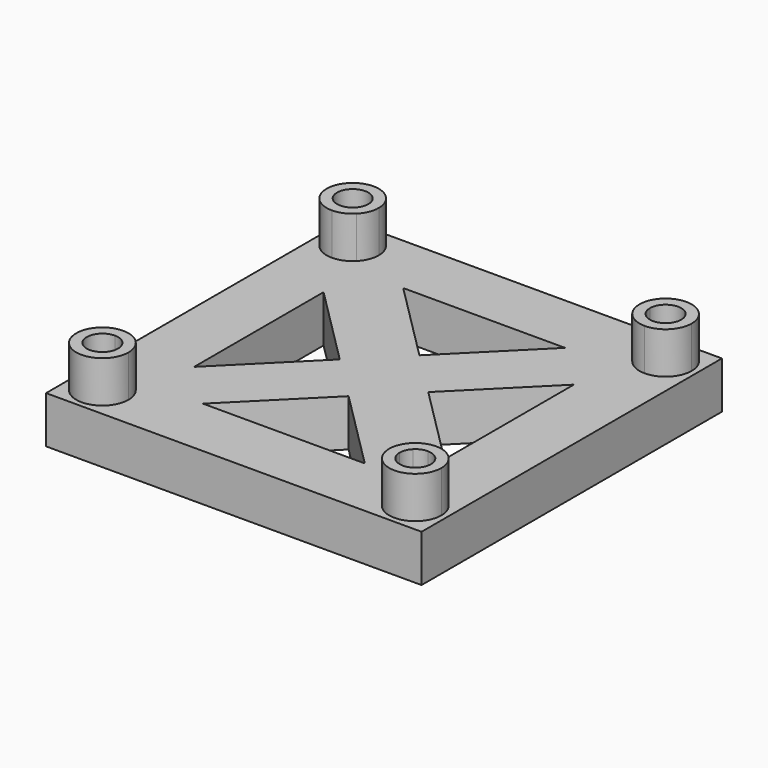
from build123d import *
from build123d import SkipClean  # not in build123d's __all__

# Parameters (mm, degrees)
F1_W     = 36
F1_H     = 36
F2_DEPTH = 4.5
F3_DEPTH = 4


with BuildPart() as f2:
    # F1 (on Top) → F2 (new body)
    with BuildSketch(Plane.XY):
        Rectangle(F1_W, F1_H)
        with BuildLine():
            ThreePointArc((-15, 12.5), (-16.767766953, 16.767766953), (-12.5, 15))
            Line((-12.5, 15), (12.5, 15))
            ThreePointArc((12.5, 15), (15, 17.5), (17.5, 15))
            ThreePointArc((17.5, 15), (16.767766953, 13.232233047), (15, 12.5))
            Line((15, 12.5), (15, -12.5))
            ThreePointArc((15, -12.5), (16.767766953, -13.232233047), (17.5, -15))
            ThreePointArc((17.5, -15), (15, -17.5), (12.5, -15))
            Line((12.5, -15), (-12.5, -15))
            ThreePointArc((-12.5, -15), (-16.767766953, -16.767766953), (-15, -12.5))
            Line((-15, -12.5), (-15, 12.5))
        make_face(mode=Mode.SUBTRACT)
        with BuildLine():
            ThreePointArc((-13.232233047, 13.232233047), (-14.0432914191, 12.6903011687), (-15, 12.5))
            Line((-15, 12.5), (-15, -12.5))
            ThreePointArc((-15, -12.5), (-14.0432914191, -12.6903011687), (-13.232233047, -13.232233047))
            Line((-13.232233047, -13.232233047), (-12, -12))
            Line((-12, -12), (-12, -7.7573593129))
            Line((-12, -7.7573593129), (-12, 7.7573593129))
            Line((-12, 7.7573593129), (-12, 12))
            Line((-12, 12), (-13.232233047, 13.232233047))
        make_face()
        with BuildLine():
            Line((12.5, 15), (-12.5, 15))
            ThreePointArc((-12.5, 15), (-12.6903011687, 14.0432914191), (-13.232233047, 13.232233047))
            Line((-13.232233047, 13.232233047), (-12, 12))
            Line((-12, 12), (-7.7573593129, 12))
            Line((-7.7573593129, 12), (7.7573593129, 12))
            Line((7.7573593129, 12), (12, 12))
            Line((12, 12), (13.232233047, 13.232233047))
            ThreePointArc((13.232233047, 13.232233047), (12.6903011687, 14.0432914191), (12.5, 15))
        make_face()
        with BuildLine():
            Line((-12, -12), (-13.232233047, -13.232233047))
            ThreePointArc((-13.232233047, -13.232233047), (-12.6903011687, -14.0432914191), (-12.5, -15))
            Line((-12.5, -15), (12.5, -15))
            ThreePointArc((12.5, -15), (12.6903011687, -14.0432914191), (13.232233047, -13.232233047))
            Line((13.232233047, -13.232233047), (12, -12))
            Line((12, -12), (7.7573593129, -12))
            Line((7.7573593129, -12), (-7.7573593129, -12))
            Line((-7.7573593129, -12), (-12, -12))
        make_face()
        with BuildLine():
            ThreePointArc((15, 12.5), (14.0432914191, 12.6903011687), (13.232233047, 13.232233047))
            Line((13.232233047, 13.232233047), (12, 12))
            Line((12, 12), (12, 7.7573593129))
            Line((12, 7.7573593129), (12, -7.7573593129))
            Line((12, -7.7573593129), (12, -12))
            Line((12, -12), (13.232233047, -13.232233047))
            ThreePointArc((13.232233047, -13.232233047), (14.0432914191, -12.6903011687), (15, -12.5))
            Line((15, -12.5), (15, 12.5))
        make_face()
        Polygon((0, 0), (-12, 12), (-12, 7.7573593129), (-4.2426406871, 0), (-2.1213203436, -2.1213203436), align=None)
        Polygon((-7.7573593129, 12), (-12, 12), (0, 0), (2.1213203436, 2.1213203436), (0, 4.2426406871), align=None)
        Polygon((2.1213203436, 2.1213203436), (0, 0), (12, -12), (12, -7.7573593129), (4.2426406871, 0), align=None)
        Polygon((12, -12), (0, 0), (-2.1213203436, -2.1213203436), (0, -4.2426406871), (7.7573593129, -12), align=None)
        Polygon((-2.1213203436, -2.1213203436), (-12, -12), (-7.7573593129, -12), (0, -4.2426406871), align=None)
        Polygon((-12, -7.7573593129), (-12, -12), (-2.1213203436, -2.1213203436), (-4.2426406871, 0), align=None)
        Polygon((2.1213203436, 2.1213203436), (12, 12), (7.7573593129, 12), (0, 4.2426406871), align=None)
        Polygon((12, 7.7573593129), (12, 12), (2.1213203436, 2.1213203436), (4.2426406871, 0), align=None)
        with BuildLine():
            Line((-13.5, 15), (-12.5, 15))
            ThreePointArc((-12.5, 15), (-16.767766953, 16.767766953), (-15, 12.5))
            Line((-15, 12.5), (-15, 13.5))
            ThreePointArc((-15, 13.5), (-16.0606601718, 16.0606601718), (-13.5, 15))
        make_face()
        with BuildLine():
            ThreePointArc((17.5, 15), (15, 17.5), (12.5, 15))
            Line((12.5, 15), (13.5, 15))
            ThreePointArc((13.5, 15), (15, 16.5), (16.5, 15))
            ThreePointArc((16.5, 15), (16.0606601718, 13.9393398282), (15, 13.5))
            Line((15, 13.5), (15, 12.5))
            ThreePointArc((15, 12.5), (16.767766953, 13.232233047), (17.5, 15))
        make_face()
        with BuildLine():
            ThreePointArc((17.5, -15), (16.767766953, -13.232233047), (15, -12.5))
            Line((15, -12.5), (15, -13.5))
            ThreePointArc((15, -13.5), (16.0606601718, -13.9393398282), (16.5, -15))
            ThreePointArc((16.5, -15), (15, -16.5), (13.5, -15))
            Line((13.5, -15), (12.5, -15))
            ThreePointArc((12.5, -15), (15, -17.5), (17.5, -15))
        make_face()
        with BuildLine():
            Line((-15, -13.5), (-15, -12.5))
            ThreePointArc((-15, -12.5), (-16.767766953, -16.767766953), (-12.5, -15))
            Line((-12.5, -15), (-13.5, -15))
            ThreePointArc((-13.5, -15), (-16.0606601718, -16.0606601718), (-15, -13.5))
        make_face()
        with BuildLine():
            Line((-15, 13.5), (-15, 12.5))
            ThreePointArc((-15, 12.5), (-14.0432914191, 12.6903011687), (-13.232233047, 13.232233047))
            Line((-13.232233047, 13.232233047), (-13.9393398282, 13.9393398282))
            ThreePointArc((-13.9393398282, 13.9393398282), (-14.4259748515, 13.6141807012), (-15, 13.5))
        make_face()
        with BuildLine():
            ThreePointArc((-13.232233047, 13.232233047), (-12.6903011687, 14.0432914191), (-12.5, 15))
            Line((-12.5, 15), (-13.5, 15))
            ThreePointArc((-13.5, 15), (-13.6141807012, 14.4259748515), (-13.9393398282, 13.9393398282))
            Line((-13.9393398282, 13.9393398282), (-13.232233047, 13.232233047))
        make_face()
        with BuildLine():
            Line((13.9393398282, 13.9393398282), (13.232233047, 13.232233047))
            ThreePointArc((13.232233047, 13.232233047), (14.0432914191, 12.6903011687), (15, 12.5))
            Line((15, 12.5), (15, 13.5))
            ThreePointArc((15, 13.5), (14.4259748515, 13.6141807012), (13.9393398282, 13.9393398282))
        make_face()
        with BuildLine():
            Line((13.5, 15), (12.5, 15))
            ThreePointArc((12.5, 15), (12.6903011687, 14.0432914191), (13.232233047, 13.232233047))
            Line((13.232233047, 13.232233047), (13.9393398282, 13.9393398282))
            ThreePointArc((13.9393398282, 13.9393398282), (13.6141807012, 14.4259748515), (13.5, 15))
        make_face()
        with BuildLine():
            ThreePointArc((13.232233047, -13.232233047), (12.6903011687, -14.0432914191), (12.5, -15))
            Line((12.5, -15), (13.5, -15))
            ThreePointArc((13.5, -15), (13.6141807012, -14.4259748515), (13.9393398282, -13.9393398282))
            Line((13.9393398282, -13.9393398282), (13.232233047, -13.232233047))
        make_face()
        with BuildLine():
            Line((15, -13.5), (15, -12.5))
            ThreePointArc((15, -12.5), (14.0432914191, -12.6903011687), (13.232233047, -13.232233047))
            Line((13.232233047, -13.232233047), (13.9393398282, -13.9393398282))
            ThreePointArc((13.9393398282, -13.9393398282), (14.4259748515, -13.6141807012), (15, -13.5))
        make_face()
        with BuildLine():
            ThreePointArc((-12.5, -15), (-12.6903011687, -14.0432914191), (-13.232233047, -13.232233047))
            Line((-13.232233047, -13.232233047), (-13.9393398282, -13.9393398282))
            ThreePointArc((-13.9393398282, -13.9393398282), (-13.6141807012, -14.4259748515), (-13.5, -15))
            Line((-13.5, -15), (-12.5, -15))
        make_face()
        with BuildLine():
            ThreePointArc((-13.232233047, -13.232233047), (-14.0432914191, -12.6903011687), (-15, -12.5))
            Line((-15, -12.5), (-15, -13.5))
            ThreePointArc((-15, -13.5), (-14.4259748515, -13.6141807012), (-13.9393398282, -13.9393398282))
            Line((-13.9393398282, -13.9393398282), (-13.232233047, -13.232233047))
        make_face()
    extrude(amount=-F2_DEPTH)

    # F1 (on Top) → F3 (join)
    with BuildSketch(Plane.XY):
        with BuildLine():
            Line((-13.5, 15), (-12.5, 15))
            ThreePointArc((-12.5, 15), (-16.767766953, 16.767766953), (-15, 12.5))
            Line((-15, 12.5), (-15, 13.5))
            ThreePointArc((-15, 13.5), (-16.0606601718, 16.0606601718), (-13.5, 15))
        make_face()
        with BuildLine():
            Line((-15, 13.5), (-15, 12.5))
            ThreePointArc((-15, 12.5), (-14.0432914191, 12.6903011687), (-13.232233047, 13.232233047))
            Line((-13.232233047, 13.232233047), (-13.9393398282, 13.9393398282))
            ThreePointArc((-13.9393398282, 13.9393398282), (-14.4259748515, 13.6141807012), (-15, 13.5))
        make_face()
        with BuildLine():
            ThreePointArc((-13.232233047, 13.232233047), (-12.6903011687, 14.0432914191), (-12.5, 15))
            Line((-12.5, 15), (-13.5, 15))
            ThreePointArc((-13.5, 15), (-13.6141807012, 14.4259748515), (-13.9393398282, 13.9393398282))
            Line((-13.9393398282, 13.9393398282), (-13.232233047, 13.232233047))
        make_face()
        with BuildLine():
            ThreePointArc((17.5, 15), (15, 17.5), (12.5, 15))
            Line((12.5, 15), (13.5, 15))
            ThreePointArc((13.5, 15), (15, 16.5), (16.5, 15))
            ThreePointArc((16.5, 15), (16.0606601718, 13.9393398282), (15, 13.5))
            Line((15, 13.5), (15, 12.5))
            ThreePointArc((15, 12.5), (16.767766953, 13.232233047), (17.5, 15))
        make_face()
        with BuildLine():
            Line((13.9393398282, 13.9393398282), (13.232233047, 13.232233047))
            ThreePointArc((13.232233047, 13.232233047), (14.0432914191, 12.6903011687), (15, 12.5))
            Line((15, 12.5), (15, 13.5))
            ThreePointArc((15, 13.5), (14.4259748515, 13.6141807012), (13.9393398282, 13.9393398282))
        make_face()
        with BuildLine():
            Line((13.5, 15), (12.5, 15))
            ThreePointArc((12.5, 15), (12.6903011687, 14.0432914191), (13.232233047, 13.232233047))
            Line((13.232233047, 13.232233047), (13.9393398282, 13.9393398282))
            ThreePointArc((13.9393398282, 13.9393398282), (13.6141807012, 14.4259748515), (13.5, 15))
        make_face()
        with BuildLine():
            Line((-15, -13.5), (-15, -12.5))
            ThreePointArc((-15, -12.5), (-16.767766953, -16.767766953), (-12.5, -15))
            Line((-12.5, -15), (-13.5, -15))
            ThreePointArc((-13.5, -15), (-16.0606601718, -16.0606601718), (-15, -13.5))
        make_face()
        with BuildLine():
            ThreePointArc((-13.232233047, -13.232233047), (-14.0432914191, -12.6903011687), (-15, -12.5))
            Line((-15, -12.5), (-15, -13.5))
            ThreePointArc((-15, -13.5), (-14.4259748515, -13.6141807012), (-13.9393398282, -13.9393398282))
            Line((-13.9393398282, -13.9393398282), (-13.232233047, -13.232233047))
        make_face()
        with BuildLine():
            ThreePointArc((-12.5, -15), (-12.6903011687, -14.0432914191), (-13.232233047, -13.232233047))
            Line((-13.232233047, -13.232233047), (-13.9393398282, -13.9393398282))
            ThreePointArc((-13.9393398282, -13.9393398282), (-13.6141807012, -14.4259748515), (-13.5, -15))
            Line((-13.5, -15), (-12.5, -15))
        make_face()
        with BuildLine():
            Line((15, -13.5), (15, -12.5))
            ThreePointArc((15, -12.5), (14.0432914191, -12.6903011687), (13.232233047, -13.232233047))
            Line((13.232233047, -13.232233047), (13.9393398282, -13.9393398282))
            ThreePointArc((13.9393398282, -13.9393398282), (14.4259748515, -13.6141807012), (15, -13.5))
        make_face()
        with BuildLine():
            ThreePointArc((13.232233047, -13.232233047), (12.6903011687, -14.0432914191), (12.5, -15))
            Line((12.5, -15), (13.5, -15))
            ThreePointArc((13.5, -15), (13.6141807012, -14.4259748515), (13.9393398282, -13.9393398282))
            Line((13.9393398282, -13.9393398282), (13.232233047, -13.232233047))
        make_face()
        with BuildLine():
            ThreePointArc((17.5, -15), (16.767766953, -13.232233047), (15, -12.5))
            Line((15, -12.5), (15, -13.5))
            ThreePointArc((15, -13.5), (16.0606601718, -13.9393398282), (16.5, -15))
            ThreePointArc((16.5, -15), (15, -16.5), (13.5, -15))
            Line((13.5, -15), (12.5, -15))
            ThreePointArc((12.5, -15), (15, -17.5), (17.5, -15))
        make_face()
    with SkipClean():  # cleaning this boolean's faces spoils the solid; the shape is the same uncleaned
        extrude(amount=F3_DEPTH)


solid = f2.part
